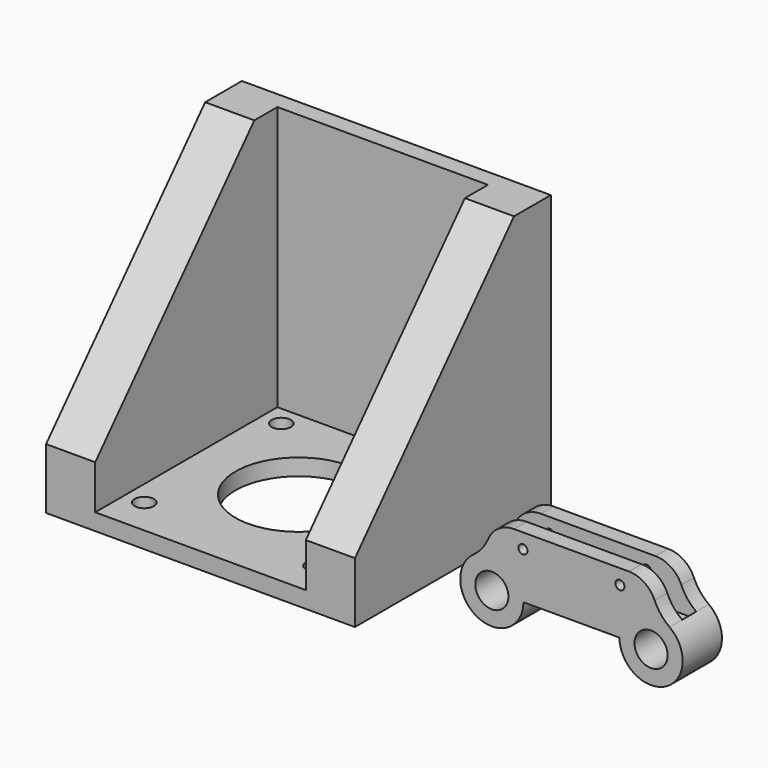
from build123d import *

# Parameters (mm, degrees)
F0_W        = 38.1
F0_H        = 38.1
F0_R        = 1.75
F0_R_2      = 11.3825570241
F0_H_2      = 3.0987125382
F1_DEPTH    = 3
F2_DEPTH    = 50.8
F4_DEPTH    = 55.88
F5_R        = 3
F5_R_2      = 0.8225607068
F6_DEPTH    = 8.89
F7_T4_DEPTH = 8.89
F7_T9_DEPTH = 8.89
F8_R        = 5.08
F9_W        = 35.5085759405
F9_H        = 3.175
F10_DEPTH   = 7.62


# Not quite as in the source:
# - a fillet or chamfer that OpenCascade refuses, or shapes differently, is made with other operations: its cross-section is extruded or revolved along the edge and cut away or added


with BuildPart() as f1:
    # F0 (on Top) → F1 (new body)
    with BuildSketch(Plane.XY):
        with Locations((-21.547248587, 4.677680321)):
            Rectangle(F0_W, F0_H)
        with Locations((-37.047248587, -10.822319679)):
            Circle(F0_R, mode=Mode.SUBTRACT)
        with Locations((-6.047248587, -10.822319679)):
            Circle(F0_R, mode=Mode.SUBTRACT)
        with Locations((-37.047248587, 20.177680321)):
            Circle(F0_R, mode=Mode.SUBTRACT)
        with Locations((-21.547248587, 4.677680321)):
            Circle(F0_R_2, mode=Mode.SUBTRACT)
        with Locations((-6.047248587, 20.177680321)):
            Circle(F0_R, mode=Mode.SUBTRACT)
        with Locations((-21.547248587, -15.9216759481)):
            Rectangle(F0_W, F0_H_2)
    extrude(amount=F1_DEPTH)

    # F0 (on Top) → F2 (join)
    with BuildSketch(Plane.XY):
        Polygon((-2.497248587, 23.727680321), (-2.497248587, -14.372319679), (-2.497248587, -17.4710322171), (6.392751413, -17.4710322171), (6.392751413, 26.8263928592), (-49.487248587, 26.8263928592), (-49.487248587, -17.4710322171), (-40.597248587, -17.4710322171), (-40.597248587, -14.372319679), (-40.597248587, 23.727680321), align=None)
    extrude(amount=F2_DEPTH)

    # F3 (on face) → F4 (cut, through all)
    with BuildSketch(Plane(origin=(-49.487248587, 0, 0), x_dir=(0, -1, 0), z_dir=(-1, 0, 0))):
        Polygon((17.4710322171, 50.8), (-18.5107886791, 50.8), (17.4710322171, 10.9709706157), align=None)
    extrude(amount=-F4_DEPTH, mode=Mode.SUBTRACT)


with BuildPart() as f6:
    # F5 (on Front) → F6 (new body)
    with BuildSketch(Plane.XZ):
        with BuildLine():
            Line((24.2974720895, 19.2513801157), (24.2974720895, 13.8756283784))
            ThreePointArc((24.2974720895, 13.8756283784), (20.256356835, 4.1195131239), (30.0124720895, 8.1606283784))
            Line((30.0124720895, 8.1606283784), (47.3918369746, 8.1606283784))
            ThreePointArc((47.3918369746, 8.1606283784), (57.1479522291, 4.1195131239), (53.1068369746, 13.8756283784))
            Line((53.1068369746, 13.8756283784), (53.1068369746, 19.2513801157))
            Line((53.1068369746, 19.2513801157), (24.2974720895, 19.2513801157))
        make_face()
        with Locations((24.2974720895, 8.1606283784)):
            Circle(F5_R, mode=Mode.SUBTRACT)
        with Locations((53.1068369746, 8.1606283784)):
            Circle(F5_R, mode=Mode.SUBTRACT)
        with Locations((29.9285501242, 16.5635042471)):
            Circle(F5_R_2, mode=Mode.SUBTRACT)
        with Locations((47.47575894, 16.5635042471)):
            Circle(F5_R_2, mode=Mode.SUBTRACT)
    extrude(amount=F6_DEPTH)

    # F7: fillet of radius 8.0943752319 on 2 edges, made by hand


with BuildPart() as f7_tool2:
    # F7_s3 → F7_t4 (new body)
    with BuildSketch(Plane.XZ):
        with BuildLine():
            ThreePointArc((24.2974720895, 19.3490122608), (23.4115248028, 15.6669643315), (20.947620726, 12.790932995))
            ThreePointArc((20.947620726, 12.790932995), (22.536927555, 13.5976963329), (24.2974720895, 13.8756283784))
            Line((24.2974720895, 13.8756283784), (24.2974720895, 19.3490122608))
        make_face()
    extrude(amount=F7_T4_DEPTH)

    split(bisect_by=Plane.XY.offset(19.2513801157), keep=Keep.BOTTOM)


with BuildPart() as f6_1:
    add(f6.part)

    # F7_t1: union F7_tool2
    add(f7_tool2.part)


with BuildPart() as f7_tool7:
    # F7_s8 → F7_t9 (new body)
    with BuildSketch(Plane.XZ):
        with BuildLine():
            ThreePointArc((56.4566883382, 12.790932995), (53.9927842613, 15.6669643315), (53.1068369746, 19.3490122608))
            Line((53.1068369746, 19.3490122608), (53.1068369746, 13.8756283784))
            ThreePointArc((53.1068369746, 13.8756283784), (54.8673815092, 13.5976963329), (56.4566883382, 12.790932995))
        make_face()
    extrude(amount=F7_T9_DEPTH)

    split(bisect_by=Plane.XY.offset(19.2513801157), keep=Keep.BOTTOM)


with BuildPart() as f6_2:
    add(f6_1.part)

    # F7_t6: union F7_tool7
    add(f7_tool7.part)

    # F8
    f8_edges = [f6_2.edges().sort_by_distance(p)[0] for p in [
        (24.296883, -4.445, 19.25138),
        (53.107426, -4.445, 19.25138),
    ]]
    fillet(f8_edges, radius=F8_R)

    # F9 (on face) → F10 (cut)
    with BuildSketch(Plane.XY.offset(19.2513801157)):
        with Locations((38.7021545321, -4.445)):
            Rectangle(F9_W, F9_H)
    extrude(amount=-F10_DEPTH, mode=Mode.SUBTRACT)


solid = Compound([f1.part, f6_2.part])
